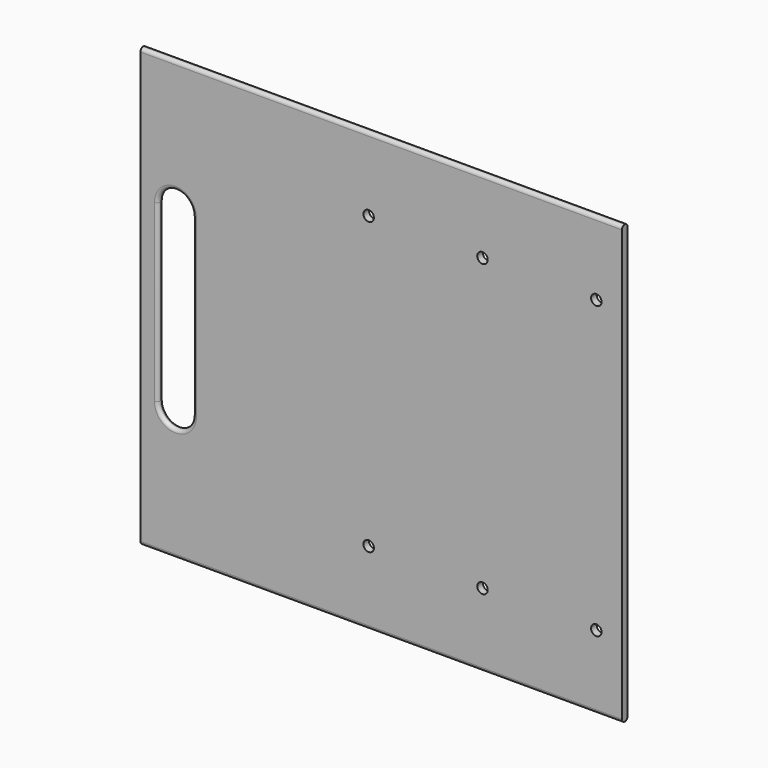
from build123d import *

# Parameters (mm, degrees)
F0_W     = 698.5
F0_H     = 635
F1_DEPTH = 10.16
F4_DEPTH = 10.161
F5_R     = 5.07999
F6_R     = 5.07999
F8_D     = 15.24


# Not quite as in the source:
# - a fillet or chamfer is up to 0.001 mm smaller than in the source, because OpenCascade refuses the exact size


with BuildPart() as f1:
    # F0 (on Front) → F1 (new body)
    with BuildSketch(Plane.XZ):
        with Locations((349.25, 317.5)):
            Rectangle(F0_W, F0_H)
    extrude(amount=F1_DEPTH)

    # F3 (on face) → F4 (cut, through all)
    with BuildSketch(Plane(origin=(0, 0, 0), x_dir=(-1, 0, 0), z_dir=(0, 1, 0))):
        with BuildLine():
            Line((-25.4, 190.5), (-25.4, 444.5))
            ThreePointArc((-25.4, 444.5), (-50.8, 469.9), (-76.2, 444.5))
            Line((-76.2, 444.5), (-76.2, 190.5))
            ThreePointArc((-76.2, 190.5), (-50.8, 165.1), (-25.4, 190.5))
        make_face()
    extrude(amount=-F4_DEPTH, mode=Mode.SUBTRACT)

    # F5 (radius 5.08 in the source; OpenCascade refuses exactly that, so slightly less here)
    f5_edges = [f1.edges().sort_by_distance(p)[0] for p in [
        (50.8, 0, 165.1),
        (76.2, -10.16, 317.5),
    ]]
    fillet(f5_edges, radius=F5_R)

    # F6 (radius 5.08 in the source; OpenCascade refuses exactly that, so slightly less here)
    f6_edges = [f1.edges().sort_by_distance(p)[0] for p in [
        (349.25, -10.16, 635),
        (349.25, 0, 635),
        (349.25, -10.16, 0),
        (349.25, 0, 0),
    ]]
    fillet(f6_edges, radius=F6_R)

    # F8 (through all)
    with Locations(Plane.XZ.offset(10.16)):
        with Locations((496.1636, 528.32), (331.0636, 528.32), (661.2636, 528.32), (661.2636, 106.68), (496.1636, 106.68), (331.0636, 106.68)):
            Hole(F8_D / 2)


solid = f1.part
